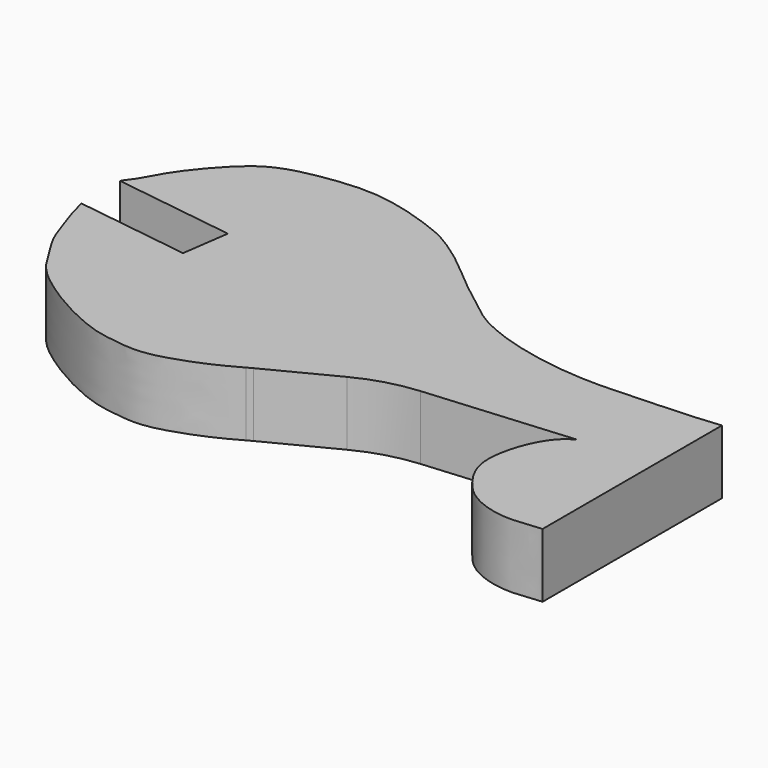
from build123d import *

# Parameters (mm, degrees)
F1_DEPTH    = 2
F2_T1_DEPTH = 2


# Not quite as in the source:
# - a fillet or chamfer that OpenCascade refuses, or shapes differently, is made with other operations: its cross-section is extruded or revolved along the edge and cut away or added


with BuildPart() as f1:
    # F0 (on Top) → F1 (new body)
    with BuildSketch(Plane.XY):
        with BuildLine():
            add(Edge.make_bspline(
                [(40.3510897258, 15.4700221217), (40.4002790123, 15.5814527788), (40.5765609139, 15.7573002366), (40.8482218334, 16.3030928425), (41.165026275, 16.7963969786), (41.6547225339, 17.4092616999), (42.2848270806, 18.0681197149), (43.024383076, 18.5173006903), (44.4482177174, 18.7966814782), (45.9437204424, 18.8740196912), (47.6474480344, 18.3309181954), (48.4387671563, 17.9801551733), (49.509499414, 17.2200044537), (50.3297293975, 16.4585906766), (51.0929989178, 15.9341416913), (51.8795462786, 15.2096607451), (53.6624560336, 14.5668169621), (55.7284365284, 14.3066111603), (57.3670281795, 14.4035559525), (59.1814684115, 14.4725478471), (59.8510897258, 14.5550060059)],
                knots=[0, 0, 0, 0, 0.0309496374, 0.0705551354, 0.1103078346, 0.1558389635, 0.2046336941, 0.2520602452, 0.3130525572, 0.3774848703, 0.4450313899, 0.4935325314, 0.5516621873, 0.6066818861, 0.6553419578, 0.7076474259, 0.7782054312, 0.8521368249, 0.9197479448, 1, 1, 1, 1], degree=3))
            Line((40.3510897258, 15.4700221217), (44.1344518025, 14.9373847717))
            Line((44.1344518025, 14.9373847717), (43.9253377729, 13.4520325163))
            Line((43.9253377729, 13.4520325163), (40.3510897258, 13.9552299289))
            add(Edge.make_bspline(
                [(40.3510897258, 13.9552299289), (40.380459386, 13.8515658436), (40.4435205062, 13.6292409687), (40.5351157189, 13.2770722669), (40.6975247029, 12.8483958981), (40.9256908997, 12.1137067954), (41.3380196001, 11.4845841437), (41.6991570459, 10.8483582383), (42.1298627814, 10.4186096604), (42.5754983268, 10.0860188118), (43.0629528901, 9.7632613692), (43.5619025736, 9.4761638561), (44.0771300551, 9.2178264046), (44.5526645941, 9.0223320072), (44.9829333509, 8.8809763782), (45.5611643118, 8.794463186), (46.382082494, 8.6943641738), (47.4820612716, 9.0173037656), (48.2852752929, 9.3514047606), (48.9644408226, 9.7399642691)],
                knots=[0, 0, 0, 0, 0.0424345091, 0.0861825949, 0.1357239466, 0.1997680722, 0.264076511, 0.3265344491, 0.3832833697, 0.4377533585, 0.4936679865, 0.5494507655, 0.6052047608, 0.6575157225, 0.7063210351, 0.761825778, 0.8279297926, 0.9033165831, 1, 1, 1, 1], degree=3))
            Line((48.9644408226, 9.7399642691), (51.9989468157, 11.3017885014))
            Line((51.9989468157, 11.3017885014), (57.5477800182, 11.7649970946))
            add(Edge.make_bspline(
                [(59.8510897258, 7.5550060059), (59.7367509498, 7.5817109742), (58.8068931658, 7.3691162235), (57.6316029399, 7.7279038973), (57.0173857229, 8.3014615446), (56.4314344596, 9.210300185), (56.556712226, 10.2745206274), (56.8370016511, 11.0042399426), (57.1435482301, 11.4671570982), (57.3374471588, 11.6295714443), (57.5477800182, 11.7649970946)],
                knots=[0, 0, 0, 0, 0.1328866261, 0.2860615837, 0.4092174064, 0.5466123808, 0.6852473434, 0.8057102912, 0.9017534238, 1, 1, 1, 1], degree=3))
            Line((59.8510897258, 7.5550060059), (59.8510897258, 14.5550060059))
        make_face()
    extrude(amount=F1_DEPTH)

    # F2: fillet of radius 5 on 2 edges, made by hand

    # F2_s2 → F2_t1 (join)
    with BuildSketch(Plane.XY):
        with BuildLine():
            ThreePointArc((52.9883634864, 11.3843835782), (52.0258606682, 11.2079480539), (51.1161547101, 10.8474258784))
            Line((51.1161547101, 10.8474258784), (51.9989468157, 11.3017885014))
            Line((51.9989468157, 11.3017885014), (52.9883634864, 11.3843835782))
        make_face()
        with BuildLine():
            ThreePointArc((49.0557948641, 9.7869831104), (48.9712088199, 9.7424196411), (48.8874903164, 9.6962469887))
            ThreePointArc((48.8874903164, 9.6962469887), (48.9259988454, 9.7180470594), (48.9644408226, 9.7399642691))
            Line((48.9644408226, 9.7399642691), (49.0557948641, 9.7869831104))
        make_face()
    extrude(amount=F2_T1_DEPTH)


solid = f1.part
